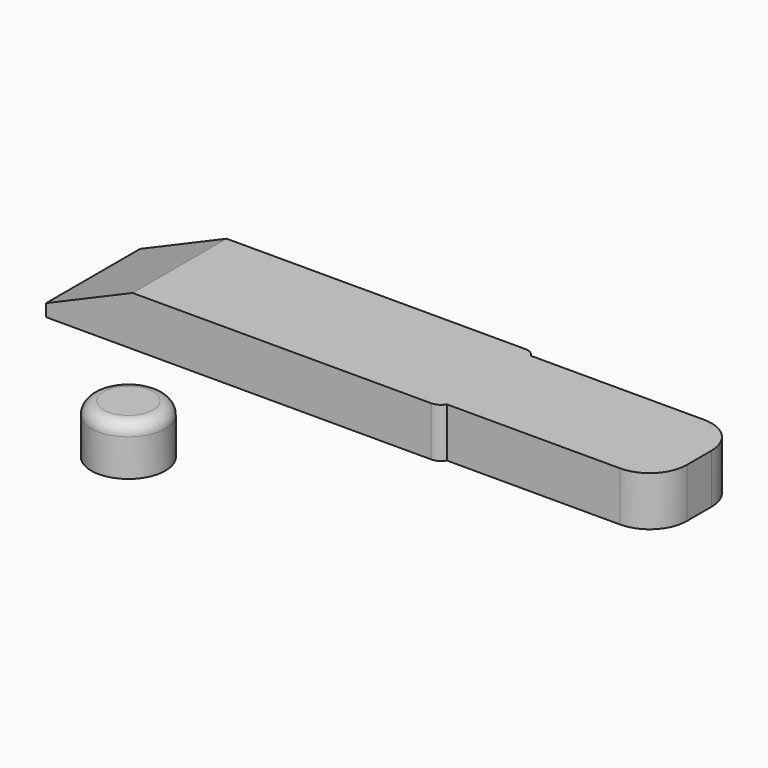
from build123d import *

# Parameters (mm, degrees)
F0_W        = 17
F0_H        = 8.5
F1_DEPTH    = 4
F0_R        = 3
F2_R        = 3
F3_SIZE2    = 7
F3_SIZE     = 3
F4_T1_DEPTH = 8.3301270189


# Not quite as in the source:
# - a fillet or chamfer that OpenCascade refuses, or shapes differently, is made with other operations: its cross-section is extruded or revolved along the edge and cut away or added


with BuildPart() as f1:
    # F0 (on Top) → F1 (new body)
    with BuildSketch(Plane.XY):
        Polygon((-16, -4.75), (16, -4.75), (16, -4.25), (16, 4.25), (16, 4.75), (-16, 4.75), align=None)
        with Locations((24.5, 0)):
            Rectangle(F0_W, F0_H)
    extrude(amount=F1_DEPTH)

    # F2
    f2_edges = [f1.edges().sort_by_distance(p)[0] for p in [
        (33, -4.25, 2),
        (33, 4.25, 2),
    ]]
    fillet(f2_edges, radius=F2_R)

    # F3
    f3_edges = [f1.edges().sort_by_distance(p)[0] for p in [
        (-16, 0, 4),
    ]]
    f3_side = f1.faces().sort_by_distance((-16, 0, 2))[0]
    chamfer(f3_edges, length=F3_SIZE, length2=F3_SIZE2, reference=f3_side)

    # F4: fillet of radius 1 on 2 edges, made by hand

    # F4_s2 → F4_t1 (cut)
    with BuildSketch(Plane.XY.offset(-2.1650635095)):
        with BuildLine():
            ThreePointArc((15.1339745962, -4.75), (15.6339745962, -4.6160254038), (16, -4.25))
            Line((16, -4.25), (16, -4.75))
            Line((16, -4.75), (15.1339745962, -4.75))
        make_face()
        with BuildLine():
            ThreePointArc((15.1339745962, 4.75), (15.6339745962, 4.6160254038), (16, 4.25))
            Line((16, 4.25), (16, 4.75))
            Line((16, 4.75), (15.1339745962, 4.75))
        make_face()
    extrude(amount=F4_T1_DEPTH, mode=Mode.SUBTRACT)


with BuildPart() as f1b:
    # F0 (on Top) → F1, piece 2 (new body)
    with BuildSketch(Plane.XY):
        with Locations((0, -16.4395216852)):
            Circle(F0_R)
    extrude(amount=F1_DEPTH)

    # F4#2: fillet of radius 1 on 1 edges, made by hand

    # F4_2_s1 → F4_2_t2 (revolve, cut)
    with BuildSketch(Plane.XZ.offset(16.4395216852)):
        with BuildLine():
            ThreePointArc((3, 3), (2.7071067812, 3.7071067812), (2, 4))
            Line((2, 4), (3, 4))
            Line((3, 4), (3, 3))
        make_face()
    revolve(axis=Axis((0, -16.4395216852, 4), (0, 0, 1)), mode=Mode.SUBTRACT)


solid = Compound([f1.part, f1b.part])
